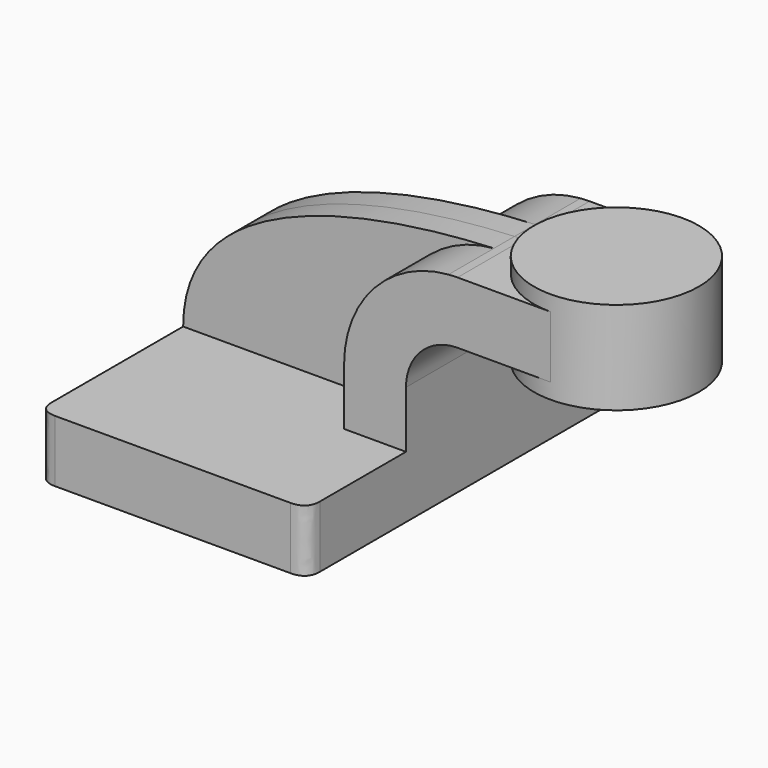
from build123d import *

# Parameters (mm, degrees)
F1_DEPTH    = 63.5
F0_W        = 25.4
F0_H        = 19.05
F2_DEPTH    = 25.4
F3_DEPTH    = 7.9375
F5_T1_DEPTH = 44.45


# Not quite as in the source:
# - a fillet or chamfer that OpenCascade refuses, or shapes differently, is made with other operations: its cross-section is extruded or revolved along the edge and cut away or added


with BuildPart() as f1:
    # F0 (on Front) → F1 (new body, symmetric)
    with BuildSketch(Plane.XZ):
        Polygon((22.225, 9.525), (-41.275, 9.525), (-41.275, -9.525), (41.275, -9.525), (41.275, 9.525), align=None)
    extrude(amount=F1_DEPTH, both=True)

    # F0 (on Front) → F2 (join, symmetric)
    with BuildSketch(Plane.XZ):
        with BuildLine():
            Line((22.225, 27.0002), (22.225, 9.525))
            Line((22.225, 9.525), (41.275, 9.525))
            Line((41.275, 9.525), (41.275, 27.0002))
            ThreePointArc((41.275, 27.0002), (45.9246798487, 38.2255201513), (57.15, 42.8752))
            Line((57.15, 42.8752), (60.325, 42.8752))
            Line((60.325, 42.8752), (60.325, 61.9252))
            Line((60.325, 61.9252), (57.15, 61.9252))
            add(Edge.make_bspline(
                [(54.3750515166, 61.8147843852), (55.3086427557, 61.8565061807), (56.2339227715, 61.893230908), (57.15, 61.9252)],
                knots=[108.9702028018, 108.9702028018, 108.9702028018, 108.9702028018, 111.5045361635, 111.5045361635, 111.5045361635, 111.5045361635], degree=3))
            ThreePointArc((54.3750515166, 61.8147843852), (31.4919534962, 50.6945089076), (22.225, 27.0002))
        make_face()
        with Locations((73.025, 52.4002)):
            Rectangle(F0_W, F0_H)
    extrude(amount=F2_DEPTH, both=True)

    # F0 (on Front) → F3 (join, symmetric)
    with BuildSketch(Plane.XZ):
        with BuildLine():
            add(Edge.make_bspline(
                [(-41.275, 9.525), (-41.275, 48.9883726548), (14.232887036, 60.0208481258), (54.3750515166, 61.8147843852)],
                knots=[0, 0, 0, 0, 108.9702028018, 108.9702028018, 108.9702028018, 108.9702028018], degree=3))
            Line((-41.275, 9.525), (22.225, 9.525))
            Line((22.225, 9.525), (22.225, 27.0002))
            ThreePointArc((22.225, 27.0002), (31.4919534962, 50.6945089076), (54.3750515166, 61.8147843852))
        make_face()
    extrude(amount=F3_DEPTH, both=True)

    # F0 (on Front) → F4 (revolve)
    with BuildSketch(Plane.XZ):
        Polygon((85.725, 66.675), (85.725, 61.9252), (85.725, 42.8752), (85.725, 38.1), (111.125, 38.1), (111.125, 66.675), align=None)
    revolve(axis=Axis((85.725, 0, 52.3875), (0, 0, 1)))

    # F5: fillet of radius 5.08 on 4 edges, made by hand

    # F5_s2 → F5_t1 (cut)
    with BuildSketch(Plane.XY.offset(-22.225)):
        with BuildLine():
            add(Edge.make_bspline(
                [(41.275, -58.42), (41.275, -63.5), (36.195, -63.5)],
                knots=[0, 0, 0, 1, 1, 1], degree=2, weights=[1, 1, 1]))
            Line((36.195, -63.5), (41.275, -63.5))
            Line((41.275, -63.5), (41.275, -58.42))
        make_face()
        with BuildLine():
            add(Edge.make_bspline(
                [(-41.275, -58.42), (-41.275, -63.5), (-36.195, -63.5)],
                knots=[0, 0, 0, 1, 1, 1], degree=2, weights=[1, 1, 1]))
            Line((-36.195, -63.5), (-41.275, -63.5))
            Line((-41.275, -63.5), (-41.275, -58.42))
        make_face()
        with BuildLine():
            add(Edge.make_bspline(
                [(41.275, 58.42), (41.275, 63.5), (36.195, 63.5)],
                knots=[0, 0, 0, 1, 1, 1], degree=2, weights=[1, 1, 1]))
            Line((36.195, 63.5), (41.275, 63.5))
            Line((41.275, 63.5), (41.275, 58.42))
        make_face()
        with BuildLine():
            add(Edge.make_bspline(
                [(-41.275, 58.42), (-41.275, 63.5), (-36.195, 63.5)],
                knots=[0, 0, 0, 1, 1, 1], degree=2, weights=[1, 1, 1]))
            Line((-36.195, 63.5), (-41.275, 63.5))
            Line((-41.275, 63.5), (-41.275, 58.42))
        make_face()
    extrude(amount=F5_T1_DEPTH, mode=Mode.SUBTRACT)


solid = f1.part
